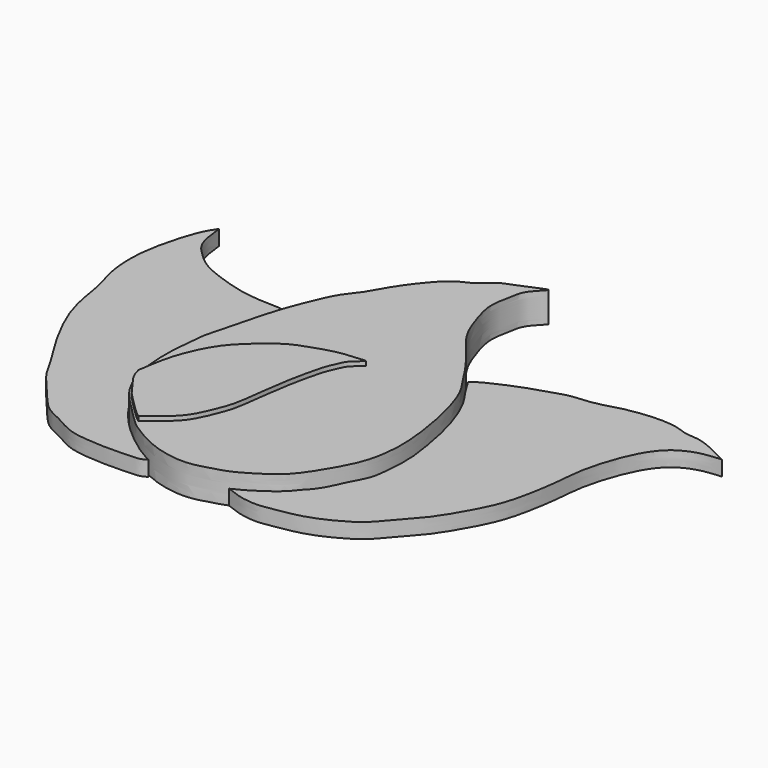
from build123d import *

# Parameters (mm, degrees)
F1_DEPTH  = 1.778
F3_DEPTH  = 3.556
F5_DEPTH  = 1.778
F10_DEPTH = 0.508


# Not quite as in the source:
# - a feature names something its author has since deleted; it is built from what else it names
# - the program builds the solid bodies; features that only make, move or delete a surface that nothing else refers to are left out


with BuildPart() as f1:
    # F0 (on Top) → F1 (new body)
    with BuildSketch(Plane.XY):
        with BuildLine():
            add(Edge.make_bspline(
                [(-34.0521857142, 24.0132473409), (-33.9219808143, 22.7885977177), (-33.6914730482, 20.6205437568), (-32.1604432516, 19.1286495269), (-30.8534845766, 17.8783061245), (-29.1550136308, 16.9850648041), (-26.8708384456, 16.1725594479), (-24.4879667806, 15.4715509571), (-21.4250164198, 15.1413445462), (-19.674372425, 15.2870244161), (-17.6439276855, 14.5293142906), (-16.9736799856, 14.3668111056), (-16.7035013437, 14.3013056368)],
                knots=[0, 0, 0, 0, 0.1259208409, 0.2229234981, 0.3138297755, 0.4080227971, 0.5138136252, 0.6236708246, 0.7423276625, 0.8348496327, 0.9334274449, 1, 1, 1, 1], degree=3))
            add(Edge.make_bspline(
                [(-34.0521857142, 24.0132473409), (-34.3284255907, 23.6049702812), (-35.0185346609, 22.5850027601), (-36.1608113995, 19.0160576566), (-36.8694139855, 15.1277566587), (-36.617444749, 11.2077409456), (-35.6075496392, 8.4588526827), (-35.1890844228, 5.149478841), (-34.2770474576, 1.7887207754), (-31.8214360912, -3.0001622678), (-29.7068115626, -6.0964363439), (-28.4397847736, -8.7138208003), (-26.2277416913, -11.0094549851), (-24.0878334221, -13.8774414641), (-22.0989196382, -14.5705707601), (-19.856915221, -16.0009476615), (-17.6525466182, -16.3788167598), (-14.3267672821, -16.55989937), (-12.3869922929, -16.3846876154), (-11.1431986408, -16.4186155672), (-10.6291924693, -16.1287594682), (-10.3948907927, -15.9966330975)],
                knots=[0, 0, 0, 0, 0.0400683032, 0.1000995938, 0.1636718905, 0.2249285605, 0.2784349913, 0.3345176463, 0.3934874099, 0.4661406769, 0.527194547, 0.5795043806, 0.6358851469, 0.694197776, 0.7393629206, 0.7891193269, 0.8365685498, 0.893665741, 0.9378845832, 0.9716856585, 1, 1, 1, 1], degree=3))
            add(Edge.make_bspline(
                [(-16.7035013437, 14.3013056368), (-17.0301024227, 13.5375401437), (-17.6776857088, 12.0231490419), (-18.3104869902, 9.8593125139), (-19.1363450149, 5.9645318319), (-19.8609016572, 3.9066748256), (-20.0251318969, 1.473598527), (-20.2227921557, -1.2863432702), (-20.2285597951, -4.1423494896), (-19.5548822163, -6.4109309928), (-18.4388920895, -9.1416317882), (-15.8732754191, -12.0505502675), (-13.8469445599, -13.7362880772), (-12.2523325508, -14.9531471987), (-11.0221872514, -15.6442263498), (-10.3948907927, -15.9966330975)],
                knots=[0, 0, 0, 0, 0.0735836342, 0.1459013296, 0.2396236317, 0.3103385219, 0.3826562325, 0.4621880484, 0.5416683878, 0.613641682, 0.6946569846, 0.7879468276, 0.8649053464, 0.9311102535, 1, 1, 1, 1], degree=3))
        make_face()
    extrude(amount=F1_DEPTH)

    # F2 (on Top) → F3 (join)
    with BuildSketch(Plane.XY):
        with BuildLine():
            add(Edge.make_bspline(
                [(-0.6725896383, 30.7766068727), (-0.7716108615, 30.9029193739), (-3.4098638922, 29.5747379513), (-5.0865264818, 29.227137572), (-6.6624901099, 27.461573806), (-8.4202687763, 26.9359859667), (-10.2777324905, 25.0996508164), (-12.4873417855, 22.1024892606), (-13.7266974683, 19.5833003681), (-15.194674433, 18.0462169446), (-16.175477689, 15.6933501794), (-16.6852662964, 14.4927188622), (-17.8374473857, 11.4493321072), (-18.4323320477, 8.784694979), (-19.2874404733, 5.6675071243), (-19.817522932, 3.8170531891), (-19.8557688712, 2.0165788724), (-20.1941526073, 0.0085288813), (-20.1450249527, -2.433946095), (-19.9944252166, -4.2362271231), (-19.6955536663, -6.1263262728), (-18.6794756963, -8.3831826724), (-17.7028739285, -9.7880422732), (-16.3777502352, -11.1262105808), (-14.9367245713, -12.5427570839), (-13.6085961653, -13.9583293072), (-11.446494912, -15.2650068721), (-9.6051252653, -16.1817872657), (-7.4816766427, -16.8019873926), (-5.0060449072, -17.034857606), (-2.7086577594, -16.3542233719), (-0.8516318469, -15.8185026313), (0.9285723481, -14.7826726905), (3.4800803963, -13.1542454132), (5.1869211598, -10.7166052062), (7.0686021516, -7.4871457798), (7.8727219116, -4.9377948969), (8.1956647667, -1.716453523), (7.837168708, 1.8623720839), (7.2225165792, 5.1759973675), (6.6178548062, 7.4325747217), (5.7094259809, 10.0012100923), (3.9734355987, 12.4816552973), (2.3535175291, 14.9646058951), (0.9734561696, 16.5443706654), (-1.167603419, 19.1377805079), (-2.1703489433, 21.9755943807), (-3.0924147257, 24.8889811765), (-2.4979613696, 27.4306626262), (-2.2814751391, 29.2634244081), (-0.5897230623, 30.6709014075), (-0.6725896383, 30.7766068727)],
                knots=[0, 0, 0, 0, 0.0212379097, 0.0401855968, 0.0591983287, 0.0765613662, 0.0973460378, 0.1227638771, 0.144518626, 0.1635899107, 0.1838264524, 0.1991169284, 0.2220722944, 0.2444262004, 0.2676605422, 0.285742356, 0.3028769358, 0.321602935, 0.341960637, 0.3594610635, 0.3774671783, 0.397858063, 0.4149684828, 0.4327126946, 0.4511979727, 0.4694417288, 0.4900161009, 0.5087951346, 0.5280389249, 0.5485433119, 0.5686468216, 0.5865832783, 0.6052140438, 0.6276004626, 0.6503250909, 0.6753498323, 0.6966674836, 0.7198305828, 0.7448346577, 0.7686825017, 0.7885531001, 0.809791013, 0.8327195934, 0.8549420417, 0.873954778, 0.8975018606, 0.9204001958, 0.942961142, 0.9635215659, 0.9822269126, 1, 1, 1, 1], degree=3))
        make_face()
    extrude(amount=F3_DEPTH)

    # F4 (on Top) → F5 (join)
    with BuildSketch(Plane.XY):
        with BuildLine():
            add(Edge.make_bspline(
                [(-0.9895847179, -15.8416330814), (-0.4249358942, -16.0641859117), (0.7510246058, -16.5276834459), (2.9580604312, -16.8463528354), (4.9777927022, -16.4273044997), (7.1623731519, -16.1193274811), (9.5287572701, -15.2930569629), (11.4951978846, -14.2325861603), (13.2708440952, -13.1041966574), (15.0735096399, -10.7060371264), (17.0081566942, -8.846495733), (19.366798954, -4.8242538721), (20.7241473891, -1.8260747887), (21.464087759, 2.0398733244), (21.7963327881, 4.5997824459), (21.9908661693, 7.4890014822), (23.0007540886, 10.8690742637), (24.0516788966, 13.2940281857), (25.602860216, 15.5695525404), (28.2399698088, 16.8454975216), (29.948997814, 16.9576697084), (30.7804513723, 17.0122422278)],
                knots=[0, 0, 0, 0, 0.0436249778, 0.0908551449, 0.1366097757, 0.1840653927, 0.2346550927, 0.2821777245, 0.3283389833, 0.3825716277, 0.4358968802, 0.5039166505, 0.5633567721, 0.6257577983, 0.6772470551, 0.7313366549, 0.7912662218, 0.8434678601, 0.8955428989, 0.9491809215, 1, 1, 1, 1], degree=3))
            add(Edge.make_bspline(
                [(30.7804513723, 17.0122422278), (30.1294623981, 17.3523547165), (28.8035237014, 18.0450981083), (26.5046387049, 18.9831384705), (25.004999975, 18.8592429646), (23.7008791306, 19.5023208868), (21.2576179243, 19.7632402123), (17.9041711653, 19.408699949), (15.859475396, 18.7592681628), (13.8603268891, 18.2956441434), (11.8462764466, 18.2710086345), (10.0491330692, 17.589719235), (7.7232004731, 16.9217382535), (5.6261809676, 16.0221768251), (3.8895099165, 15.2437616337), (3.1857400761, 14.7335924), (2.8715927619, 14.505864121)],
                knots=[0, 0, 0, 0, 0.0750840913, 0.1529317793, 0.2124773762, 0.2703479172, 0.3483746308, 0.4402766667, 0.5136335457, 0.5841856112, 0.6541882895, 0.7229866625, 0.8004876985, 0.8766815575, 0.9449533707, 1, 1, 1, 1], degree=3))
            add(Edge.make_bspline(
                [(2.8715927619, 14.505864121), (3.1629086632, 14.0022142037), (3.801552015, 12.8980771827), (5.3690597508, 10.8049284413), (6.4468290231, 8.1121791606), (7.3378340142, 5.2043219041), (7.9735482219, 1.5515708229), (8.3123811205, -0.9380409084), (8.1170189745, -3.9863048097), (7.8351396528, -6.1062116532), (6.6552763788, -7.9668004109), (5.9473013035, -9.9236114769), (4.5794923073, -11.7905972849), (2.8165083242, -13.0850778385), (1.4536393713, -14.616606539), (-0.134956548, -15.4131246214), (-0.9895847179, -15.8416330814)],
                knots=[0, 0, 0, 0, 0.0611551259, 0.1340685984, 0.2109405617, 0.2907696961, 0.3773231318, 0.4501743102, 0.5283908831, 0.594615916, 0.6605568102, 0.7260387581, 0.7943546768, 0.8609093524, 0.9251724217, 1, 1, 1, 1], degree=3))
        make_face()
    extrude(amount=F5_DEPTH)

    # F9 (on face) → F10 (join)
    with BuildSketch(Plane.XY.offset(3.556)):
        with BuildLine():
            add(Edge.make_bspline(
                [(-13.8124432415, -13.206818141), (-13.4785445061, -12.945251137), (-12.7338188139, -12.361853695), (-11.1013208399, -11.0642136034), (-10.0487586546, -9.6980126409), (-9.2130778254, -7.8369800814), (-8.5082214321, -5.9791666315), (-8.2131274762, -4.2389660769), (-7.6978518379, 0.0845494466), (-7.2181536627, 2.3673554824), (-6.6983098083, 4.9483241764), (-5.8699638884, 6.7511842253), (-5.4439830463, 7.570066596), (-3.9738265008, 8.5817813239), (-4.5709050166, 8.4893728876), (-4.7964593396, 8.454464376)],
                knots=[0, 0, 0, 0, 0.0664797412, 0.1482760072, 0.2235119453, 0.3047896017, 0.3835499444, 0.4606169328, 0.5783653889, 0.66846815, 0.7602764258, 0.8388707219, 0.8978401613, 0.9614077669, 1, 1, 1, 1], degree=3))
            add(Edge.make_bspline(
                [(-4.7964593396, 8.454464376), (-5.5896829647, 8.4093484745), (-7.1947814664, 8.3180558508), (-9.5921268698, 7.5869800641), (-12.2726687897, 6.6562724638), (-14.6281413684, 4.6626452955), (-16.9294416097, 2.4962823066), (-18.6198759159, -1.1520660439), (-19.2174796746, -3.8250778305), (-19.4389209726, -5.3216158894), (-19.542939961, -6.024593953)],
                knots=[0, 0, 0, 0, 0.1147127113, 0.2321226892, 0.3567642068, 0.4861159898, 0.6189201731, 0.7669697266, 0.8905372507, 1, 1, 1, 1], degree=3))
            add(Edge.make_bspline(
                [(-19.542939961, -6.024593953), (-19.4227126705, -6.4483335807), (-19.1703129818, -7.3379132233), (-18.1362292735, -8.6141763549), (-17.2802112063, -9.9533130155), (-16.0224817472, -11.1257189713), (-14.4024670663, -12.7877080471), (-13.9661996664, -13.0976007383), (-13.8124432415, -13.206818141)],
                knots=[0, 0, 0, 0, 0.1572478744, 0.3301190136, 0.4996298713, 0.6822918096, 0.8880281324, 1, 1, 1, 1], degree=3))
        make_face()
    extrude(amount=F10_DEPTH)


solid = f1.part
